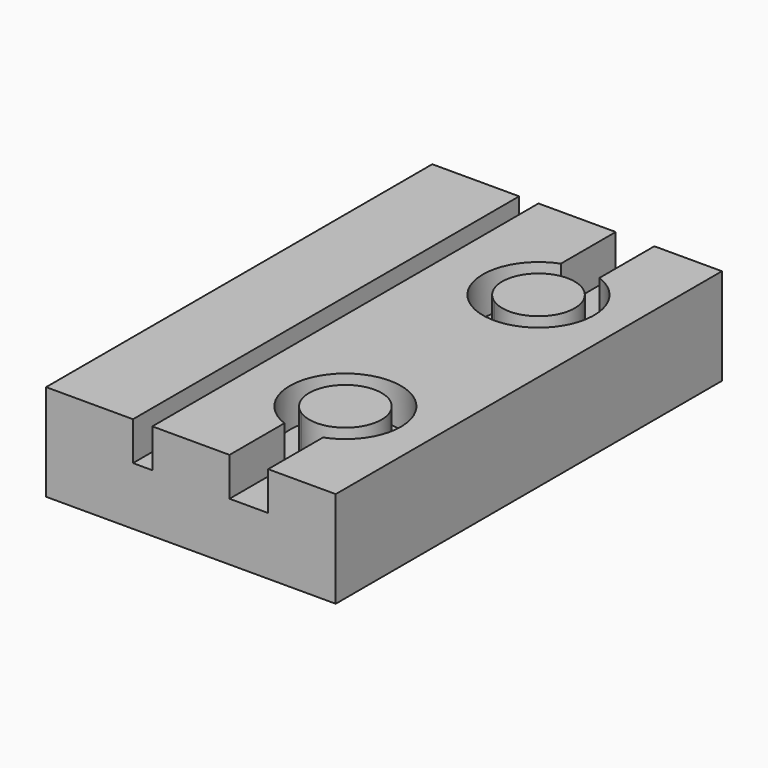
from build123d import *

# Parameters (mm, degrees)
F0_W      = 60
F0_H      = 100
F1_DEPTH  = 10
F2_W      = 4
F2_H      = 8
F2_W_2    = 8
F3_DEPTH  = 100.001
F5_W      = 8
F5_H      = 8
F6_DEPTH  = 25
F8_DEPTH  = 8
F10_DEPTH = 8


# Not quite as in the source:
# - a feature names something its author has since deleted; it is built from what else it names


with BuildPart() as f1:
    # F0 (on Top) → F1 (new body, symmetric)
    with BuildSketch(Plane.XY):
        Rectangle(F0_W, F0_H)
    extrude(amount=F1_DEPTH, both=True)

    # F2 (on face) → F3 (cut, through all)
    with BuildSketch(Plane.XZ.offset(50)):
        with Locations((-10, 6)):
            Rectangle(F2_W, F2_H)
        with Locations((12, 6)):
            Rectangle(F2_W_2, F2_H)
    extrude(amount=-F3_DEPTH, mode=Mode.SUBTRACT)

    # F5 (on Front) → F6 (join, symmetric)
    with BuildSketch(Plane.XZ):
        with Locations((12, 6)):
            Rectangle(F5_W, F5_H)
    extrude(amount=F6_DEPTH, both=True)

    # F7 (on face) → F8 (cut, through all)
    with BuildSketch(Plane.XY.offset(10)):
        with BuildLine():
            ThreePointArc((8, 35.7819293264), (0.5, 25), (8, 14.2180706736))
            Line((8, 14.2180706736), (8, 18.6557112298))
            ThreePointArc((8, 18.6557112298), (4.5, 25), (8, 31.3442887702))
            Line((8, 31.3442887702), (8, 35.7819293264))
        make_face()
        with BuildLine():
            ThreePointArc((8, -31.3442887702), (4.5, -25), (8, -18.6557112298))
            Line((8, -18.6557112298), (8, -14.2180706736))
            ThreePointArc((8, -14.2180706736), (0.5, -25), (8, -35.7819293264))
            Line((8, -35.7819293264), (8, -31.3442887702))
        make_face()
        with BuildLine():
            Line((8, 18.6557112298), (8, 14.2180706736))
            ThreePointArc((8, 14.2180706736), (18.5669627683, 15.5593962058), (23.5, 25))
            ThreePointArc((23.5, 25), (18.5669627683, 34.4406037942), (8, 35.7819293264))
            Line((8, 35.7819293264), (8, 31.3442887702))
            ThreePointArc((8, 31.3442887702), (15.6228441865, 31.5669627683), (19.5, 25))
            ThreePointArc((19.5, 25), (15.6228441865, 18.4330372317), (8, 18.6557112298))
        make_face()
        with BuildLine():
            ThreePointArc((8, -18.6557112298), (15.6228441865, -18.4330372317), (19.5, -25))
            ThreePointArc((19.5, -25), (15.6228441865, -31.5669627683), (8, -31.3442887702))
            Line((8, -31.3442887702), (8, -35.7819293264))
            ThreePointArc((8, -35.7819293264), (18.5669627683, -34.4406037942), (23.5, -25))
            ThreePointArc((23.5, -25), (18.5669627683, -15.5593962058), (8, -14.2180706736))
            Line((8, -14.2180706736), (8, -18.6557112298))
        make_face()
    extrude(amount=-F8_DEPTH, mode=Mode.SUBTRACT)

    # F9 (on face) → F10 (join, through all)
    with BuildSketch(Plane.XY.offset(10)):
        with BuildLine():
            ThreePointArc((8, -31.3442887702), (15.6228441865, -31.5669627683), (19.5, -25))
            ThreePointArc((19.5, -25), (15.6228441865, -18.4330372317), (8, -18.6557112298))
            Line((8, -18.6557112298), (8, -31.3442887702))
        make_face()
        with BuildLine():
            Line((8, 31.3442887702), (8, 18.6557112298))
            ThreePointArc((8, 18.6557112298), (15.6228441865, 18.4330372317), (19.5, 25))
            ThreePointArc((19.5, 25), (15.6228441865, 31.5669627683), (8, 31.3442887702))
        make_face()
        with BuildLine():
            ThreePointArc((8, 31.3442887702), (4.5, 25), (8, 18.6557112298))
            Line((8, 18.6557112298), (8, 31.3442887702))
        make_face()
    extrude(amount=-F10_DEPTH)


solid = f1.part
